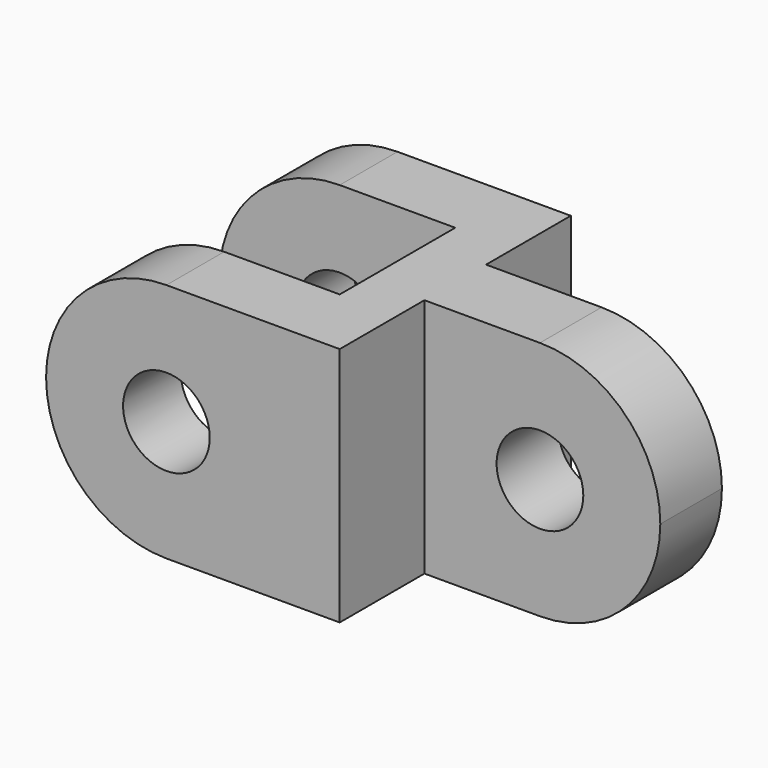
from build123d import *

# Parameters (mm, degrees)
F0_W     = 110
F0_H     = 60
F1_DEPTH = 50
F2_W     = 49
F2_H     = 22
F2_W_2   = 48.9966
F2_H_2   = 21.9964
F2_H_3   = 30
F3_DEPTH = 50
F4_R     = 24.99999
F5_R     = 9
F5_R_2   = 9.0043
F6_DEPTH = 25.07751
F7_DEPTH = 58.2571


# Not quite as in the source:
# - a fillet or chamfer is up to 0.001 mm smaller than in the source, because OpenCascade refuses the exact size


with BuildPart() as f1:
    # F0 (on Top) → F1 (new body)
    with BuildSketch(Plane.XY):
        with Locations((-0.4379451275, 12.3298443558)):
            Rectangle(F0_W, F0_H)
    extrude(amount=F1_DEPTH)

    # F2 (on Top) → F3 (cut)
    with BuildSketch(Plane.XY):
        with Locations((30.0620548725, -6.6701556442)):
            Rectangle(F2_W, F2_H)
        with Locations((30.0637548725, 31.3316443558)):
            Rectangle(F2_W_2, F2_H_2)
        with Locations((-30.9379451275, 12.3298443558)):
            Rectangle(F2_W, F2_H_3)
    extrude(amount=F3_DEPTH, mode=Mode.SUBTRACT)

    # F4 (radius 25 in the source; OpenCascade refuses exactly that, so slightly less here)
    f4_edges = [f1.edges().sort_by_distance(p)[0] for p in [
        (-55.437945, 34.829844, 50),
        (-55.437945, 34.829844, 0),
        (-55.437945, -10.170156, 50),
        (-55.437945, -10.170156, 0),
        (54.562055, 12.331644, 50),
        (54.562055, 12.331644, 0),
    ]]
    fillet(f4_edges, radius=F4_R)

    # F5 (on Front) → F6 (cut, symmetric)
    with BuildSketch(Plane.XZ):
        with Locations((-30.4379451275, 25)):
            Circle(F5_R)
        with Locations((29.5620548725, 25.0064)):
            Circle(F5_R_2)
    extrude(amount=F6_DEPTH, both=True, mode=Mode.SUBTRACT)

    # F5 (on Front) → F7 (cut)
    with BuildSketch(Plane.XZ):
        with Locations((-30.4379451275, 25)):
            Circle(F5_R)
        with Locations((29.5620548725, 25.0064)):
            Circle(F5_R_2)
    extrude(amount=-F7_DEPTH, mode=Mode.SUBTRACT)


solid = f1.part
